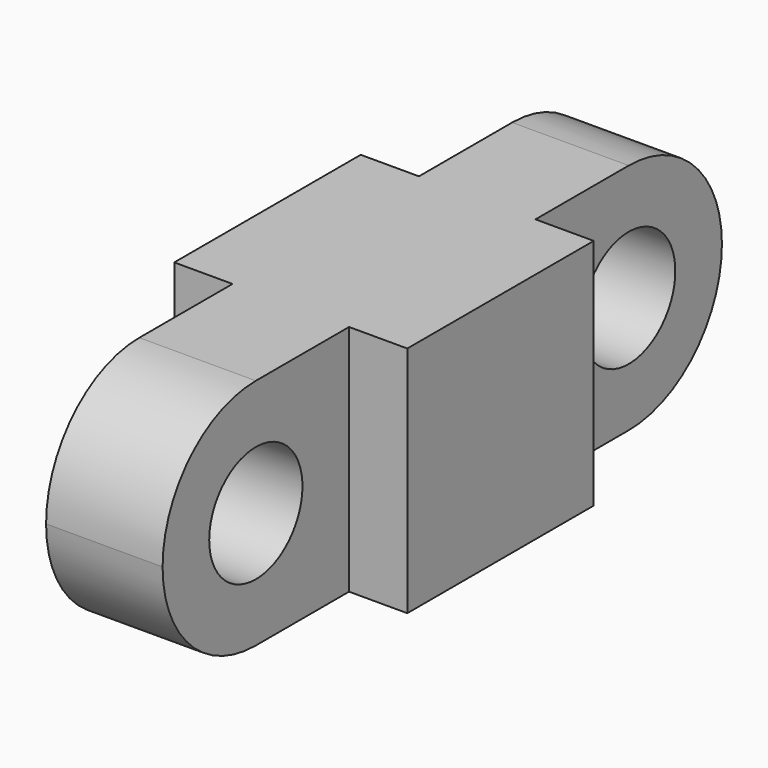
from build123d import *

# Parameters (mm, degrees)
F1_DEPTH = 40
F2_R     = 10
F3_DEPTH = 20
F4_R     = 10
F5_DEPTH = 20
F6_R     = 20
F7_R     = 19.99999
F8_R     = 20
F9_R     = 19.99999


# Not quite as in the source:
# - a fillet or chamfer is up to 0.001 mm smaller than in the source, because OpenCascade refuses the exact size


with BuildPart() as f1:
    # F0 (on Top) → F1 (new body)
    with BuildSketch(Plane.XY):
        Polygon((10, 40), (10, 0), (30, 0), (30, 40), (40, 40), (40, 80), (30, 80), (30, 120), (10, 120), (10, 80), (0, 80), (0, 40), align=None)
    extrude(amount=F1_DEPTH)

    # F2 (on face) → F3 (cut)
    with BuildSketch(Plane(origin=(10, 0, 0), x_dir=(0, -1, 0), z_dir=(-1, 0, 0))):
        with Locations((-100, 20)):
            Circle(F2_R)
    extrude(amount=-F3_DEPTH, mode=Mode.SUBTRACT)

    # F4 (on face) → F5 (cut)
    with BuildSketch(Plane(origin=(10, 0, 0), x_dir=(0, -1, 0), z_dir=(-1, 0, 0))):
        with Locations((-20, 20)):
            Circle(F4_R)
    extrude(amount=-F5_DEPTH, mode=Mode.SUBTRACT)

    # F6
    f6_edges = [f1.edges().sort_by_distance(p)[0] for p in [
        (20, 0, 40),
    ]]
    fillet(f6_edges, radius=F6_R)

    # F7 (radius 20 in the source; OpenCascade refuses exactly that, so slightly less here)
    f7_edges = [f1.edges().sort_by_distance(p)[0] for p in [
        (20, 0, 0),
    ]]
    fillet(f7_edges, radius=F7_R)

    # F8
    f8_edges = [f1.edges().sort_by_distance(p)[0] for p in [
        (20, 120, 40),
    ]]
    fillet(f8_edges, radius=F8_R)

    # F9 (radius 20 in the source; OpenCascade refuses exactly that, so slightly less here)
    f9_edges = [f1.edges().sort_by_distance(p)[0] for p in [
        (20, 120, 0),
    ]]
    fillet(f9_edges, radius=F9_R)


solid = f1.part
